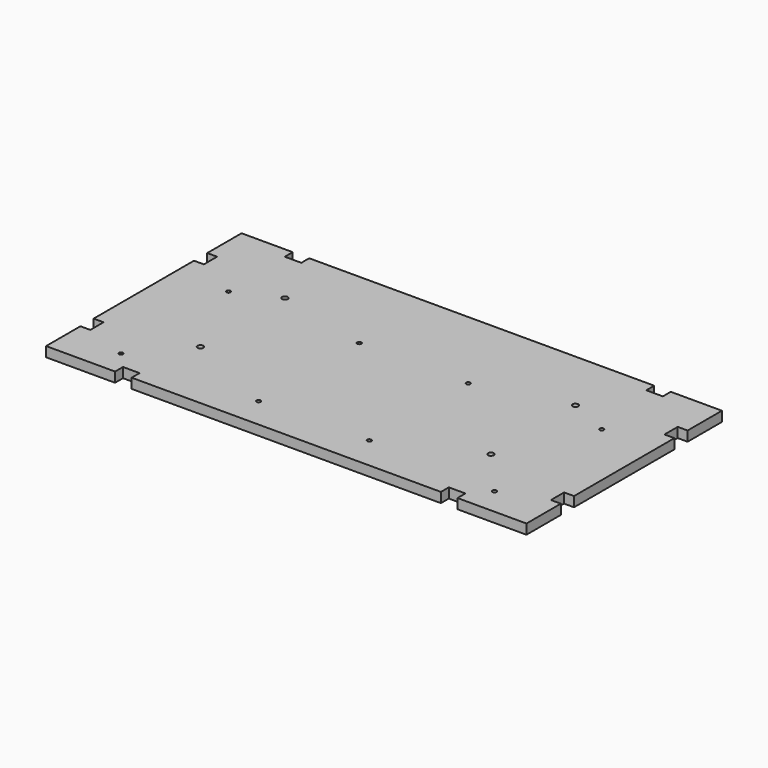
from build123d import *

# Parameters (mm, degrees)
F0_R     = 1.25
F0_R_2   = 1.75
F1_DEPTH = 6


# Not quite as in the source:
# - a feature names something its author has since deleted; it is built from what else it names


with BuildPart() as f1:
    # F0 (on Top) → F1 (new body)
    with BuildSketch(Plane.XY):
        Polygon((145.5019380654, -28.2040820618), (145.5019380654, 47.7959179382), (139.5019380654, 47.7959179382), (139.5019380654, 57.7961117593), (145.5019380654, 57.7961117593), (145.4994183911, 83.7961116372), (114.4994185367, 83.7931074102), (114.5, 77.7931074384), (104.5, 77.7931074384), (104.5, 83.793107429), (0, 83.793107429), (-104.5, 83.793107429), (-104.5, 77.7931074384), (-114.5, 77.7931074384), (-114.4994185367, 83.7931074102), (-145.4994183911, 83.7961116372), (-145.5019380654, 57.7961117593), (-139.5019380654, 57.7961117593), (-139.5019380654, 47.7959179382), (-145.5019380654, 47.7959179382), (-145.5019380654, -28.2040820618), (-139.5019380654, -28.2040820618), (-139.5019380654, -38.2040820618), (-145.5019380652, -38.2041248082), (-145.5019380652, -64.2040820618), (-103.7128691326, -64.2040817458), (-103.7128691326, -58.2040817458), (-93.6722421218, -58.2040816699), (-93.6722421218, -64.2042880704), (-4.2916e-06, -64.2042880704), (93.6722421218, -64.2042880704), (93.6722421218, -58.2040816699), (103.7128691326, -58.2040817458), (103.7128691326, -64.2040817458), (145.5019380652, -64.2040820618), (145.5019380652, -38.2041248082), (139.5019380654, -38.2040820618), (139.5019380654, -28.2040820618), align=None)
        with Locations((-113.03, -48.0000058421)):
            Circle(F0_R, mode=Mode.SUBTRACT)
        with Locations((-31.75, -45.4600058421)):
            Circle(F0_R, mode=Mode.SUBTRACT)
        with Locations((-88, -19.2042880704)):
            Circle(F0_R_2, mode=Mode.SUBTRACT)
        with Locations((34.29, -44.1900058421)):
            Circle(F0_R, mode=Mode.SUBTRACT)
        with Locations((113.03, -47.8810681991)):
            Circle(F0_R, mode=Mode.SUBTRACT)
        with Locations((88, -19.2042880704)):
            Circle(F0_R_2, mode=Mode.SUBTRACT)
        with Locations((-113.03, 33.2799941579)):
            Circle(F0_R, mode=Mode.SUBTRACT)
        with Locations((-88, 44.7957119296)):
            Circle(F0_R_2, mode=Mode.SUBTRACT)
        with Locations((-31.75, 30.7399941579)):
            Circle(F0_R, mode=Mode.SUBTRACT)
        with Locations((34.29, 30.7399941579)):
            Circle(F0_R, mode=Mode.SUBTRACT)
        with Locations((88, 44.7957119296)):
            Circle(F0_R_2, mode=Mode.SUBTRACT)
        with Locations((113.03, 33.3989318009)):
            Circle(F0_R, mode=Mode.SUBTRACT)
    extrude(amount=F1_DEPTH)


solid = f1.part
